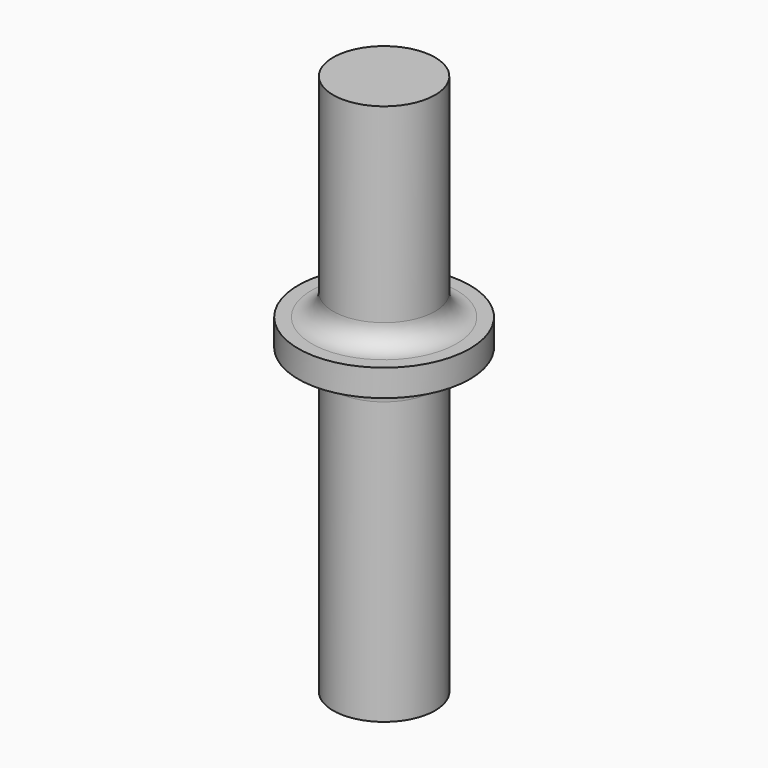
from build123d import *

# Parameters (mm, degrees)
F0_R          = 9.5
F1_DEPTH      = 42
F1_DEPTH_BACK = 59
F2_R          = 16
F3_DEPTH      = 2.5
F3_DEPTH_BACK = 2.5
F4_R          = 4


with BuildPart() as f1:
    # F0 (on Top) → F1 (new body, two sides)
    with BuildSketch(Plane.XY) as f1_sk:
        Circle(F0_R)
    extrude(amount=F1_DEPTH)
    extrude(f1_sk.sketch, amount=-F1_DEPTH_BACK)

    # F2 (on Top) → F3 (join, two sides)
    with BuildSketch(Plane.XY) as f3_sk:
        Circle(F2_R)
    extrude(amount=F3_DEPTH)
    extrude(f3_sk.sketch, amount=-F3_DEPTH_BACK)

    # F4
    f4_edges = [f1.edges().sort_by_distance(p)[0] for p in [
        (-9.5, 0, -2.5),
        (-9.5, 0, 2.5),
    ]]
    fillet(f4_edges, radius=F4_R)


solid = f1.part
